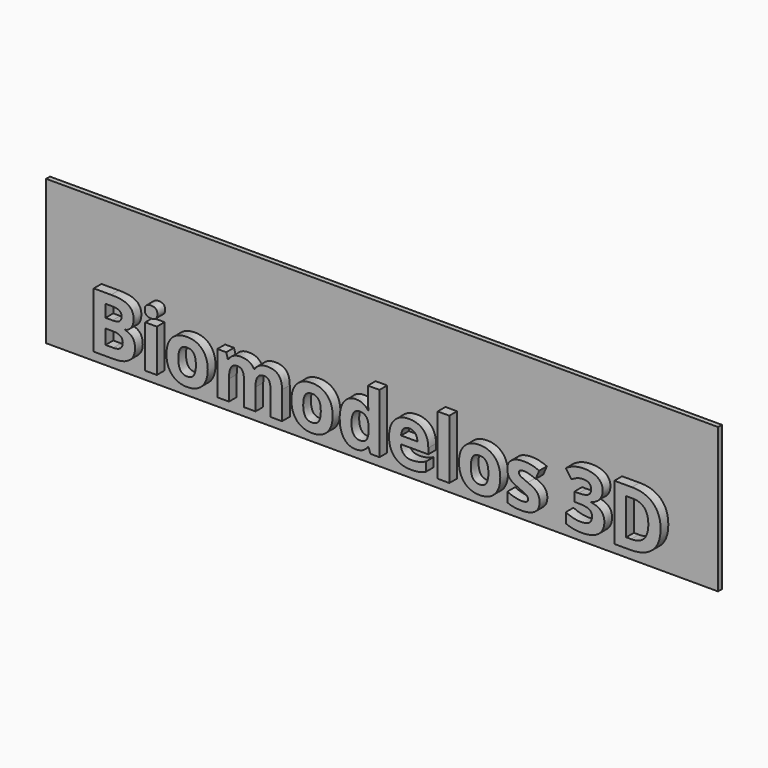
from build123d import *

# Parameters (mm, degrees)
F0_TEXT_SIZE = 8.0862533693
F1_DEPTH     = 1
F2_W         = 69.6470110773
F2_H         = 15
F3_DEPTH     = 0.5


# Not quite as in the source:
# - Text() gives the source's letters only with a copy of the font that has no kerning and outlines rounded to 1/6400 em; it was checked with that copy


with BuildPart() as f1:
    # F0 (on Front) → F1 (new body)
    with BuildSketch(Plane.XZ):
        with Locations((0, 0)):
            Text('Biomodelos 3D', F0_TEXT_SIZE, font='Open Sans', font_style=FontStyle.BOLD, text_align=(TextAlign.LEFT, TextAlign.BOTTOM))
    extrude(amount=F1_DEPTH)

    # F2 (on Front) → F3 (join)
    with BuildSketch(Plane.XZ):
        with Locations((29.8103419482, 6)):
            Rectangle(F2_W, F2_H)
    extrude(amount=-F3_DEPTH)


solid = f1.part
